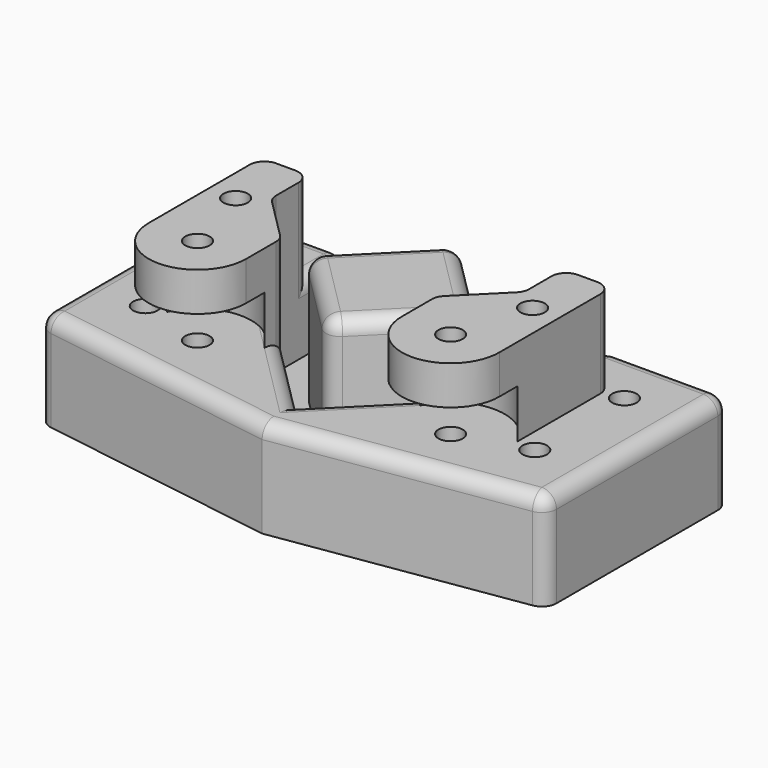
from build123d import *

# Parameters (mm, degrees)
F3_DEPTH      = 32
F0_R          = 2.5
F4_DEPTH      = 6
F5_DEPTH      = 20
F6_DEPTH      = 38
F2_R          = 11
F7_DEPTH      = 10
F8_T1_DEPTH   = 35.1066017178
F8_T3_DEPTH   = 18.6032957828
F8_T5_DEPTH   = 18.6032957828
F8_T7_DEPTH   = 18.6032957828
F8_T9_DEPTH   = 18.6032957828
F8_T11_DEPTH  = 23
F8_T13_DEPTH  = 21.1066017178
F8_T15_DEPTH  = 25.5
F8_T17_DEPTH  = 11
F8_T19_DEPTH  = 24.5
F8_T21_DEPTH  = 23.4343921757
F8_T23_DEPTH  = 7.1853823869
F8_T25_DEPTH  = 20
F8_T27_DEPTH  = 41.4262431297
F8_T29_DEPTH  = 62.7880288816
F8_T31_DEPTH  = 62.7880288816
F8_T33_DEPTH  = 20
F8_T35_DEPTH  = 52
F8_S39_W      = 3
F8_S39_H      = 3
F8_T40_DEPTH  = 3
F8_T46_DEPTH  = 3
F8_S51_W      = 3
F8_S51_H      = 3
F8_T52_DEPTH  = 3
F8_S57_W      = 3
F8_S57_H      = 3
F8_T58_DEPTH  = 3
F8_S63_W      = 3
F8_S63_H      = 3
F8_T64_DEPTH  = 3
F8_S69_W      = 3
F8_S69_H      = 3
F8_T70_DEPTH  = 3
F8_T76_DEPTH  = 3
F8_S81_W      = 3
F8_S81_H      = 3
F8_T82_DEPTH  = 3
F8_T88_DEPTH  = 3
F8_S93_W      = 3
F8_S93_H      = 3
F8_T94_DEPTH  = 3
F8_T100_DEPTH = 30.127416998
F8_S101_R     = 11
F8_T102_DEPTH = 18
F8_T107_DEPTH = 30.127416998
F8_T112_DEPTH = 30.127416998
F8_S113_R     = 11
F8_T114_DEPTH = 18
F8_T119_DEPTH = 30.127416998
F8_T124_DEPTH = 30.127416998
F8_S126_R     = 11
F8_T127_DEPTH = 18
F8_T131_DEPTH = 30.127416998
F8_S133_R     = 11
F8_T134_DEPTH = 18
F8_T139_DEPTH = 30.127416998
F8_S140_R     = 11
F8_T141_DEPTH = 18
F8_T145_DEPTH = 24.2132034356
F8_T152_DEPTH = 37.627416998
F8_T156_DEPTH = 37.627416998
F8_T163_DEPTH = 24.2132034356
F8_T167_DEPTH = 30.127416998
F8_S169_R     = 11
F8_T170_DEPTH = 18
F8_T176_DEPTH = 14.6853823869
F8_T180_DEPTH = 33
F8_T187_DEPTH = 33
F8_T191_DEPTH = 14.6853823869
F8_T198_DEPTH = 59.5
F8_T202_DEPTH = 18.5
F8_T209_DEPTH = 59.5
F8_T213_DEPTH = 18.5


# Not quite as in the source:
# - a fillet or chamfer that OpenCascade refuses, or shapes differently, is made with other operations: its cross-section is extruded or revolved along the edge and cut away or added


with BuildPart() as f3:
    # F0 (on Top) → F3 (new body)
    with BuildSketch(Plane.XY):
        Polygon((17.3971572875, -21.7171572875), (0, -4.32), (-17.3971572875, -21.7171572875), (0, -39.1143145751), align=None)
    extrude(amount=F3_DEPTH)

    # F0 (on Top) → F4 (join)
    with BuildSketch(Plane.XY):
        Polygon((26, 0), (0, 0), (-26, 0), (-26, -10.1853823869), (-26, -20.1853823869), (-16, -30.1853823869), (0, -46.1853823869), (16, -30.1853823869), (26, -20.1853823869), (26, -10.1853823869), align=None)
        with Locations((-21, -12)):
            Circle(F0_R, mode=Mode.SUBTRACT)
        Polygon((-17.3971572875, -21.7171572875), (0, -4.32), (17.3971572875, -21.7171572875), (0, -39.1143145751), align=None, mode=Mode.SUBTRACT)
        with Locations((21, -12)):
            Circle(F0_R, mode=Mode.SUBTRACT)
    extrude(amount=F4_DEPTH)

    # F0 (on Top) → F5 (join)
    with BuildSketch(Plane.XY):
        with BuildLine():
            Line((52, 0), (26, 0))
            Line((26, 0), (26, -10.1853823869))
            Line((26, -10.1853823869), (36, -10.1853823869))
            Line((36, -10.1853823869), (36, -39.1143145751))
            ThreePointArc((36, -39.1143145751), (26, -49.1143145751), (16, -39.1143145751))
            Line((16, -39.1143145751), (16, -30.1853823869))
            Line((16, -30.1853823869), (0, -46.1853823869))
            Line((0, -46.1853823869), (-16, -30.1853823869))
            Line((-16, -30.1853823869), (-16, -39.1143145751))
            ThreePointArc((-16, -39.1143145751), (-26, -49.1143145751), (-36, -39.1143145751))
            Line((-36, -39.1143145751), (-36, -10.1853823869))
            Line((-36, -10.1853823869), (-26, -10.1853823869))
            Line((-26, -10.1853823869), (-26, 0))
            Line((-26, 0), (-52, 0))
            Line((-52, 0), (-52, -47))
            Line((-52, -47), (0, -55))
            Line((0, -55), (52, -47))
            Line((52, -47), (52, 0))
        make_face()
        with Locations((-40, -35)):
            Circle(F0_R, mode=Mode.SUBTRACT)
        with Locations((40, -35)):
            Circle(F0_R, mode=Mode.SUBTRACT)
        with Locations((-40, -12)):
            Circle(F0_R, mode=Mode.SUBTRACT)
        with Locations((40, -12)):
            Circle(F0_R, mode=Mode.SUBTRACT)
    extrude(amount=F5_DEPTH)

    # F0 (on Top) → F6 (join)
    with BuildSketch(Plane.XY):
        with BuildLine():
            Line((-26, -20.1853823869), (-26, -10.1853823869))
            Line((-26, -10.1853823869), (-36, -10.1853823869))
            Line((-36, -10.1853823869), (-36, -39.1143145751))
            ThreePointArc((-36, -39.1143145751), (-26, -49.1143145751), (-16, -39.1143145751))
            Line((-16, -39.1143145751), (-16, -30.1853823869))
            Line((-16, -30.1853823869), (-26, -20.1853823869))
        make_face()
        with Locations((-26, -39.1143145751)):
            Circle(F0_R, mode=Mode.SUBTRACT)
        with Locations((-30.5, -23.6853823869)):
            Circle(F0_R, mode=Mode.SUBTRACT)
        with BuildLine():
            Line((36, -10.1853823869), (26, -10.1853823869))
            Line((26, -10.1853823869), (26, -20.1853823869))
            Line((26, -20.1853823869), (16, -30.1853823869))
            Line((16, -30.1853823869), (16, -39.1143145751))
            ThreePointArc((16, -39.1143145751), (26, -49.1143145751), (36, -39.1143145751))
            Line((36, -39.1143145751), (36, -10.1853823869))
        make_face()
        with Locations((26, -39.1143145751)):
            Circle(F0_R, mode=Mode.SUBTRACT)
        with Locations((30.5, -23.6853823869)):
            Circle(F0_R, mode=Mode.SUBTRACT)
    extrude(amount=F6_DEPTH)

    # F2 (on offset) → F7 (cut)
    with BuildSketch(Plane.XY.offset(20)):
        with Locations((-26, -39)):
            Circle(F2_R)
        with Locations((26, -39)):
            Circle(F2_R)
    extrude(amount=F7_DEPTH, mode=Mode.SUBTRACT)

    # F8: fillet of radius 3 on 33 edges, made by hand

    # F8_s2 → F8_t1 (join)
    with BuildSketch(Plane.XY.offset(2.8933982822)):
        with BuildLine():
            ThreePointArc((-26, -18.9427416998), (-25.7716385975, -20.0907919969), (-25.1213203436, -21.0640620434))
            Line((-25.1213203436, -21.0640620434), (-26, -20.1853823869))
            Line((-26, -20.1853823869), (-26, -18.9427416998))
        make_face()
        with BuildLine():
            ThreePointArc((25.1213203436, -21.0640620434), (25.7716385975, -20.0907919969), (26, -18.9427416998))
            Line((26, -18.9427416998), (26, -20.1853823869))
            Line((26, -20.1853823869), (25.1213203436, -21.0640620434))
        make_face()
    extrude(amount=F8_T1_DEPTH)

    # F8_s4 → F8_t3 (cut)
    with BuildSketch(Plane(origin=(4.2813203436, -4.2813203436, 0), x_dir=(0, 0, 1), z_dir=(0.7071067812, -0.7071067812, 0))):
        with BuildLine():
            ThreePointArc((32, 24.6579970775), (31.1213203436, 26.779317421), (29, 27.6579970775))
            Line((29, 27.6579970775), (32, 27.6579970775))
            Line((32, 27.6579970775), (32, 24.6579970775))
        make_face()
    extrude(amount=F8_T3_DEPTH, mode=Mode.SUBTRACT)

    # F8_s6 → F8_t5 (cut)
    with BuildSketch(Plane(origin=(17.435836944, -17.435836944, 0), x_dir=(0, 0, 1), z_dir=(-0.7071067812, 0.7071067812, 0))):
        with BuildLine():
            ThreePointArc((29, -3.0547012947), (31.1213203436, -3.9333809512), (32, -6.0547012947))
            Line((32, -6.0547012947), (32, -3.0547012947))
            Line((32, -3.0547012947), (29, -3.0547012947))
        make_face()
    extrude(amount=F8_T5_DEPTH, mode=Mode.SUBTRACT)

    # F8_s8 → F8_t7 (cut)
    with BuildSketch(Plane(origin=(-4.2813203436, -4.2813203436, 0), x_dir=(0, 0, 1), z_dir=(-0.7071067812, -0.7071067812, 0))):
        with BuildLine():
            ThreePointArc((29, -3.0547012947), (31.1213203436, -3.9333809512), (32, -6.0547012947))
            Line((32, -6.0547012947), (32, -3.0547012947))
            Line((32, -3.0547012947), (29, -3.0547012947))
        make_face()
    extrude(amount=F8_T7_DEPTH, mode=Mode.SUBTRACT)

    # F8_s10 → F8_t9 (cut)
    with BuildSketch(Plane(origin=(-17.435836944, -17.435836944, 0), x_dir=(0, 0, 1), z_dir=(0.7071067812, 0.7071067812, 0))):
        with BuildLine():
            ThreePointArc((32, 24.6579970775), (31.1213203436, 26.779317421), (29, 27.6579970775))
            Line((29, 27.6579970775), (32, 27.6579970775))
            Line((32, 27.6579970775), (32, 24.6579970775))
        make_face()
    extrude(amount=F8_T9_DEPTH, mode=Mode.SUBTRACT)

    # F8_s12 → F8_t11 (cut)
    with BuildSketch(Plane.XY.offset(6)):
        with BuildLine():
            ThreePointArc((2.1213203436, -36.9929942315), (0, -37.8716738879), (-2.1213203436, -36.9929942315))
            Line((-2.1213203436, -36.9929942315), (0, -39.1143145751))
            Line((0, -39.1143145751), (2.1213203436, -36.9929942315))
        make_face()
        with BuildLine():
            ThreePointArc((15.275836944, -19.595836944), (16.1545166004, -21.7171572875), (15.275836944, -23.8384776311))
            Line((15.275836944, -23.8384776311), (17.3971572875, -21.7171572875))
            Line((17.3971572875, -21.7171572875), (15.275836944, -19.595836944))
        make_face()
        with BuildLine():
            ThreePointArc((2.1213203436, -6.4413203436), (0, -5.5626406871), (-2.1213203436, -6.4413203436))
            Line((-2.1213203436, -6.4413203436), (0, -4.32))
            Line((0, -4.32), (2.1213203436, -6.4413203436))
        make_face()
        with BuildLine():
            ThreePointArc((-15.275836944, -19.595836944), (-16.1545166004, -21.7171572875), (-15.275836944, -23.8384776311))
            Line((-15.275836944, -23.8384776311), (-17.3971572875, -21.7171572875))
            Line((-17.3971572875, -21.7171572875), (-15.275836944, -19.595836944))
        make_face()
    extrude(amount=F8_T11_DEPTH, mode=Mode.SUBTRACT)

    # F8_s14 → F8_t13 (cut)
    with BuildSketch(Plane.XY.offset(20)):
        with BuildLine():
            ThreePointArc((16.8786796564, -29.3067027305), (16.2283614025, -30.2799727769), (16, -31.428023074))
            Line((16, -31.428023074), (16, -30.1853823869))
            Line((16, -30.1853823869), (16.8786796564, -29.3067027305))
        make_face()
        with BuildLine():
            ThreePointArc((-16.8786796564, -29.3067027305), (-16.2283614025, -30.2799727769), (-16, -31.428023074))
            Line((-16, -31.428023074), (-16, -30.1853823869))
            Line((-16, -30.1853823869), (-16.8786796564, -29.3067027305))
        make_face()
    extrude(amount=F8_T13_DEPTH, mode=Mode.SUBTRACT)

    # F8_s16 → F8_t15 (cut)
    with BuildSketch(Plane.XY.offset(20)):
        with BuildLine():
            ThreePointArc((-26, -13.1853823869), (-26.8786796564, -11.0640620434), (-29, -10.1853823869))
            Line((-29, -10.1853823869), (-26, -10.1853823869))
            Line((-26, -10.1853823869), (-26, -13.1853823869))
        make_face()
        with BuildLine():
            ThreePointArc((26, -13.1853823869), (26.8786796564, -11.0640620434), (29, -10.1853823869))
            Line((29, -10.1853823869), (26, -10.1853823869))
            Line((26, -10.1853823869), (26, -13.1853823869))
        make_face()
        with BuildLine():
            ThreePointArc((-33, -10.1853823869), (-35.1213203436, -11.0640620434), (-36, -13.1853823869))
            Line((-36, -13.1853823869), (-36, -10.1853823869))
            Line((-36, -10.1853823869), (-33, -10.1853823869))
        make_face()
        with BuildLine():
            ThreePointArc((33, -10.1853823869), (35.1213203436, -11.0640620434), (36, -13.1853823869))
            Line((36, -13.1853823869), (36, -10.1853823869))
            Line((36, -10.1853823869), (33, -10.1853823869))
        make_face()
    extrude(amount=F8_T15_DEPTH, mode=Mode.SUBTRACT)

    # F8_s18 → F8_t17 (cut)
    with BuildSketch(Plane.XY.offset(6)):
        with BuildLine():
            ThreePointArc((29, 0), (26.8786796564, -0.8786796564), (26, -3))
            Line((26, -3), (26, 0))
            Line((26, 0), (29, 0))
        make_face()
        with BuildLine():
            ThreePointArc((-29, 0), (-26.8786796564, -0.8786796564), (-26, -3))
            Line((-26, -3), (-26, 0))
            Line((-26, 0), (-29, 0))
        make_face()
    extrude(amount=F8_T17_DEPTH, mode=Mode.SUBTRACT)

    # F8_s20 → F8_t19 (cut)
    with BuildSketch(Plane.XY.offset(-7.5)):
        with BuildLine():
            ThreePointArc((-49, 0), (-51.1213203436, -0.8786796564), (-52, -3))
            Line((-52, -3), (-52, 0))
            Line((-52, 0), (-49, 0))
        make_face()
        with BuildLine():
            ThreePointArc((49, 0), (51.1213203436, -0.8786796564), (52, -3))
            Line((52, -3), (52, 0))
            Line((52, 0), (49, 0))
        make_face()
    extrude(amount=F8_T19_DEPTH, mode=Mode.SUBTRACT)

    # F8_s22 → F8_t21 (cut)
    with BuildSketch(Plane.XY.offset(-6.4343921757)):
        with BuildLine():
            ThreePointArc((-52, -44.4262431297), (-51.2768964248, -46.3796357351), (-49.4561715528, -47.3913582227))
            Line((-49.4561715528, -47.3913582227), (-52, -47))
            Line((-52, -47), (-52, -44.4262431297))
        make_face()
        with BuildLine():
            ThreePointArc((52, -44.4262431297), (51.2768964248, -46.3796357351), (49.4561715528, -47.3913582227))
            Line((49.4561715528, -47.3913582227), (52, -47))
            Line((52, -47), (52, -44.4262431297))
        make_face()
    extrude(amount=F8_T21_DEPTH, mode=Mode.SUBTRACT)

    # F8_s24 → F8_t23 (cut)
    with BuildSketch(Plane.XZ.offset(3)):
        with BuildLine():
            ThreePointArc((26, 17), (26.8786796564, 19.1213203436), (29, 20))
            Line((29, 20), (26, 20))
            Line((26, 20), (26, 17))
        make_face()
        with BuildLine():
            ThreePointArc((-26, 17), (-26.8786796564, 19.1213203436), (-29, 20))
            Line((-29, 20), (-26, 20))
            Line((-26, 20), (-26, 17))
        make_face()
    extrude(amount=F8_T23_DEPTH, mode=Mode.SUBTRACT)

    # F8_s26 → F8_t25 (cut)
    with BuildSketch(Plane.YZ.offset(29)):
        with BuildLine():
            ThreePointArc((0, 17), (-0.8786796564, 19.1213203436), (-3, 20))
            Line((-3, 20), (0, 20))
            Line((0, 20), (0, 17))
        make_face()
    extrude(amount=F8_T25_DEPTH, mode=Mode.SUBTRACT)

    # F8_s28 → F8_t27 (cut)
    with BuildSketch(Plane.XZ.offset(3)):
        with BuildLine():
            ThreePointArc((49, 20), (51.1213203436, 19.1213203436), (52, 17))
            Line((52, 17), (52, 20))
            Line((52, 20), (49, 20))
        make_face()
        with BuildLine():
            ThreePointArc((-49, 20), (-51.1213203436, 19.1213203436), (-52, 17))
            Line((-52, 17), (-52, 20))
            Line((-52, 20), (-49, 20))
        make_face()
    extrude(amount=F8_T27_DEPTH, mode=Mode.SUBTRACT)

    # F8_s30 → F8_t29 (cut)
    with BuildSketch(Plane(origin=(-20.8676350988, -3.2104053998, 0), x_dir=(0, 0, 1), z_dir=(0.9883716977, 0.1520571843, 0))):
        with BuildLine():
            ThreePointArc((20, 51.3604433708), (19.1213203436, 53.4817637143), (17, 54.3604433708))
            Line((17, 54.3604433708), (20, 54.3604433708))
            Line((20, 54.3604433708), (20, 51.3604433708))
        make_face()
    extrude(amount=F8_T29_DEPTH, mode=Mode.SUBTRACT)

    # F8_s32 → F8_t31 (cut)
    with BuildSketch(Plane(origin=(-41.190275599, 6.3369654768, 0), x_dir=(0, 0, 1), z_dir=(0.9883716977, -0.1520571843, 0))):
        with BuildLine():
            ThreePointArc((20, 51.3604433708), (19.1213203436, 53.4817637143), (17, 54.3604433708))
            Line((17, 54.3604433708), (20, 54.3604433708))
            Line((20, 54.3604433708), (20, 51.3604433708))
        make_face()
    extrude(amount=F8_T31_DEPTH, mode=Mode.SUBTRACT)

    # F8_s34 → F8_t33 (cut)
    with BuildSketch(Plane.YZ.offset(-49)):
        with BuildLine():
            ThreePointArc((0, 17), (-0.8786796564, 19.1213203436), (-3, 20))
            Line((-3, 20), (0, 20))
            Line((0, 20), (0, 17))
        make_face()
    extrude(amount=F8_T33_DEPTH, mode=Mode.SUBTRACT)

    # F8_s36 → F8_t35 (cut)
    with BuildSketch(Plane.YZ.offset(-26)):
        with BuildLine():
            ThreePointArc((-3, 6), (-0.8786796564, 5.1213203436), (0, 3))
            Line((0, 3), (0, 6))
            Line((0, 6), (-3, 6))
        make_face()
    extrude(amount=F8_T35_DEPTH, mode=Mode.SUBTRACT)


with BuildPart() as f8_tool38:
    # F8_s39 → F8_t40 (new body)
    with BuildSketch(Plane(origin=(4.2813203436, -4.2813203436, 0), x_dir=(0, 0, 1), z_dir=(-0.7071067812, 0.7071067812, 0))):
        with Locations((30.5, -26.1579970775)):
            Rectangle(F8_S39_W, F8_S39_H)
    extrude(amount=F8_T40_DEPTH)

    # F8_s41 → F8_t42 (revolve, cut)
    with BuildSketch(Plane(origin=(-13.1545166004, -21.7171572875, 29), x_dir=(0.5, 0.5, -0.7071067812), z_dir=(0.5, 0.5, 0.7071067812))):
        with BuildLine():
            ThreePointArc((0, -3), (3, 0), (0, 3))
            Line((0, 3), (0, -3))
        make_face()
    revolve(axis=Axis((-13.1545166004, -21.7171572875, 29), (-0.7071067812, 0.7071067812, 0)), mode=Mode.SUBTRACT)


with BuildPart() as f3_1:
    add(f3.part)

    # F8_t37: cut F8_tool38
    add(f8_tool38.part, mode=Mode.SUBTRACT)


with BuildPart() as f8_tool44:
    # F8_s45 → F8_t46 (new body)
    with BuildSketch(Plane.XY.offset(29)):
        Polygon((0, -34.8716738879), (2.1213203436, -36.9929942315), (0, -39.1143145751), (-2.1213203436, -36.9929942315), align=None)
    extrude(amount=F8_T46_DEPTH)

    # F8_s47 → F8_t48 (revolve, cut)
    with BuildSketch(Plane(origin=(0, -34.8716738879, 29), x_dir=(0, 1, 0), z_dir=(1, 0, 0))):
        with BuildLine():
            ThreePointArc((0, -3), (3, 0), (0, 3))
            Line((0, 3), (0, -3))
        make_face()
    revolve(axis=Axis((0, -34.8716738879, 29), (0, 0, 1)), mode=Mode.SUBTRACT)


with BuildPart() as f3_2:
    add(f3_1.part)

    # F8_t43: cut F8_tool44
    add(f8_tool44.part, mode=Mode.SUBTRACT)


with BuildPart() as f8_tool50:
    # F8_s51 → F8_t52 (new body)
    with BuildSketch(Plane(origin=(-4.2813203436, -4.2813203436, 0), x_dir=(0, 0, 1), z_dir=(0.7071067812, 0.7071067812, 0))):
        with Locations((30.5, 26.1579970775)):
            Rectangle(F8_S51_W, F8_S51_H)
    extrude(amount=F8_T52_DEPTH)

    # F8_s53 → F8_t54 (revolve, cut)
    with BuildSketch(Plane(origin=(13.1545166004, -21.7171572875, 29), x_dir=(-0.5, 0.5, -0.7071067812), z_dir=(0.5, -0.5, -0.7071067812))):
        with BuildLine():
            ThreePointArc((0, -3), (3, 0), (0, 3))
            Line((0, 3), (0, -3))
        make_face()
    revolve(axis=Axis((13.1545166004, -21.7171572875, 29), (0.7071067812, 0.7071067812, 0)), mode=Mode.SUBTRACT)


with BuildPart() as f3_3:
    add(f3_2.part)

    # F8_t49: cut F8_tool50
    add(f8_tool50.part, mode=Mode.SUBTRACT)


with BuildPart() as f8_tool56:
    # F8_s57 → F8_t58 (new body)
    with BuildSketch(Plane(origin=(-4.2813203436, -4.2813203436, 0), x_dir=(0, 0, 1), z_dir=(0.7071067812, 0.7071067812, 0))):
        with Locations((30.5, 4.5547012947)):
            Rectangle(F8_S57_W, F8_S57_H)
    extrude(amount=F8_T58_DEPTH)

    # F8_s59 → F8_t60 (revolve, cut)
    with BuildSketch(Plane(origin=(0, -8.5626406871, 29), x_dir=(0.5, -0.5, -0.7071067812), z_dir=(0.5, -0.5, 0.7071067812))):
        with BuildLine():
            ThreePointArc((0, -3), (3, 0), (0, 3))
            Line((0, 3), (0, -3))
        make_face()
    revolve(axis=Axis((0, -8.5626406871, 29), (0.7071067812, 0.7071067812, 0)), mode=Mode.SUBTRACT)


with BuildPart() as f3_4:
    add(f3_3.part)

    # F8_t55: cut F8_tool56
    add(f8_tool56.part, mode=Mode.SUBTRACT)


with BuildPart() as f8_tool62:
    # F8_s63 → F8_t64 (new body)
    with BuildSketch(Plane.XZ.offset(3)):
        with Locations((27.5, 18.5)):
            Rectangle(F8_S63_W, F8_S63_H)
    extrude(amount=-F8_T64_DEPTH)

    # F8_s65 → F8_t66 (revolve, cut)
    with BuildSketch(Plane(origin=(29, -3, 17), x_dir=(0.7071067812, 0, -0.7071067812), z_dir=(0.7071067812, 0, 0.7071067812))):
        with BuildLine():
            ThreePointArc((0, -3), (3, 0), (0, 3))
            Line((0, 3), (0, -3))
        make_face()
    revolve(axis=Axis((29, -3, 17), (0, 1, 0)), mode=Mode.SUBTRACT)


with BuildPart() as f3_5:
    add(f3_4.part)

    # F8_t61: cut F8_tool62
    add(f8_tool62.part, mode=Mode.SUBTRACT)


with BuildPart() as f8_tool68:
    # F8_s69 → F8_t70 (new body)
    with BuildSketch(Plane.YZ.offset(-49)):
        with Locations((-1.5, 18.5)):
            Rectangle(F8_S69_W, F8_S69_H)
    extrude(amount=-F8_T70_DEPTH)

    # F8_s71 → F8_t72 (revolve, cut)
    with BuildSketch(Plane(origin=(-49, -3, 17), x_dir=(0, -0.7071067812, -0.7071067812), z_dir=(0, 0.7071067812, -0.7071067812))):
        with BuildLine():
            ThreePointArc((0, -3), (3, 0), (0, 3))
            Line((0, 3), (0, -3))
        make_face()
    revolve(axis=Axis((-49, -3, 17), (-1, 0, 0)), mode=Mode.SUBTRACT)


with BuildPart() as f3_6:
    add(f3_5.part)

    # F8_t67: cut F8_tool68
    add(f8_tool68.part, mode=Mode.SUBTRACT)


with BuildPart() as f8_tool74:
    # F8_s75 → F8_t76 (new body)
    with BuildSketch(Plane.XY.offset(17)):
        Polygon((-49, -44.4262431297), (-52, -44.4262431297), (-52, -47), (-49.4561715528, -47.3913582227), align=None)
    extrude(amount=F8_T76_DEPTH)

    # F8_s77 → F8_t78 (revolve, cut)
    with BuildSketch(Plane(origin=(-49, -44.4262431297, 17), x_dir=(0.7589654749, 0.6511308685, 0), z_dir=(0.6511308685, -0.7589654749, 0))):
        with BuildLine():
            ThreePointArc((0, -3), (3, 0), (0, 3))
            Line((0, 3), (0, -3))
        make_face()
    revolve(axis=Axis((-49, -44.4262431297, 17), (0, 0, 1)), mode=Mode.SUBTRACT)


with BuildPart() as f3_7:
    add(f3_6.part)

    # F8_t73: cut F8_tool74
    add(f8_tool74.part, mode=Mode.SUBTRACT)


with BuildPart() as f8_tool80:
    # F8_s81 → F8_t82 (new body)
    with BuildSketch(Plane.YZ.offset(49)):
        with Locations((-1.5, 18.5)):
            Rectangle(F8_S81_W, F8_S81_H)
    extrude(amount=F8_T82_DEPTH)

    # F8_s83 → F8_t84 (revolve, cut)
    with BuildSketch(Plane(origin=(49, -3, 17), x_dir=(0, -0.7071067812, -0.7071067812), z_dir=(0, -0.7071067812, 0.7071067812))):
        with BuildLine():
            ThreePointArc((0, -3), (3, 0), (0, 3))
            Line((0, 3), (0, -3))
        make_face()
    revolve(axis=Axis((49, -3, 17), (1, 0, 0)), mode=Mode.SUBTRACT)


with BuildPart() as f3_8:
    add(f3_7.part)

    # F8_t79: cut F8_tool80
    add(f8_tool80.part, mode=Mode.SUBTRACT)


with BuildPart() as f8_tool86:
    # F8_s87 → F8_t88 (new body)
    with BuildSketch(Plane.XY.offset(17)):
        Polygon((49, -44.4262431297), (52, -44.4262431297), (52, -47), (49.4561715528, -47.3913582227), align=None)
    extrude(amount=F8_T88_DEPTH)

    # F8_s89 → F8_t90 (revolve, cut)
    with BuildSketch(Plane(origin=(49, -44.4262431297, 17), x_dir=(-0.7589654749, 0.6511308685, 0), z_dir=(0.6511308685, 0.7589654749, 0))):
        with BuildLine():
            ThreePointArc((0, -3), (3, 0), (0, 3))
            Line((0, 3), (0, -3))
        make_face()
    revolve(axis=Axis((49, -44.4262431297, 17), (0, 0, 1)), mode=Mode.SUBTRACT)


with BuildPart() as f3_9:
    add(f3_8.part)

    # F8_t85: cut F8_tool86
    add(f8_tool86.part, mode=Mode.SUBTRACT)


with BuildPart() as f8_tool92:
    # F8_s93 → F8_t94 (new body)
    with BuildSketch(Plane.YZ.offset(-29)):
        with Locations((-1.5, 18.5)):
            Rectangle(F8_S93_W, F8_S93_H)
    extrude(amount=F8_T94_DEPTH)

    # F8_s95 → F8_t96 (revolve, cut)
    with BuildSketch(Plane(origin=(-29, -3, 17), x_dir=(0, -0.7071067812, -0.7071067812), z_dir=(0, -0.7071067812, 0.7071067812))):
        with BuildLine():
            ThreePointArc((0, -3), (3, 0), (0, 3))
            Line((0, 3), (0, -3))
        make_face()
    revolve(axis=Axis((-29, -3, 17), (1, 0, 0)), mode=Mode.SUBTRACT)


with BuildPart() as f3_10:
    add(f3_9.part)

    # F8_t91: cut F8_tool92
    add(f8_tool92.part, mode=Mode.SUBTRACT)


with BuildPart() as f8_tool98:
    # F8_s99 → F8_t100 (new body)
    with BuildSketch(Plane(origin=(-1.7893903346, -1.7893903346, 0), x_dir=(0, 0, 1), z_dir=(-0.7071067812, -0.7071067812, 0))):
        with BuildLine():
            ThreePointArc((17, -32.6579970775), (19.1213203436, -33.5366767339), (20, -35.6579970775))
            Line((20, -35.6579970775), (20, -32.6579970775))
            Line((20, -32.6579970775), (17, -32.6579970775))
        make_face()
    extrude(amount=F8_T100_DEPTH)

    # F8_s101 → F8_t102 (intersect, symmetric)
    with BuildSketch(Plane.XY.offset(18.5)):
        with Locations((26, -39)):
            Circle(F8_S101_R)
    extrude(amount=F8_T102_DEPTH, both=True, mode=Mode.INTERSECT)

    split(bisect_by=Plane.YZ.offset(16), keep=Keep.TOP)


with BuildPart() as f3_11:
    add(f3_10.part)

    # F8_t97: cut F8_tool98
    add(f8_tool98.part, mode=Mode.SUBTRACT)


with BuildPart() as f8_tool105:
    # F8_s106 → F8_t107 (new body)
    with BuildSketch(Plane(origin=(-1.7893903346, -1.7893903346, 0), x_dir=(0, 0, 1), z_dir=(-0.7071067812, -0.7071067812, 0))):
        with BuildLine():
            ThreePointArc((17, -32.6579970775), (19.1213203436, -33.5366767339), (20, -35.6579970775))
            Line((20, -35.6579970775), (20, -32.6579970775))
            Line((20, -32.6579970775), (17, -32.6579970775))
        make_face()
    extrude(amount=F8_T107_DEPTH)

    split(bisect_by=Plane.YZ.offset(16), keep=Keep.BOTTOM)


with BuildPart() as f3_12:
    add(f3_11.part)

    # F8_t104: cut F8_tool105
    add(f8_tool105.part, mode=Mode.SUBTRACT)


with BuildPart() as f8_tool110:
    # F8_s111 → F8_t112 (new body)
    with BuildSketch(Plane(origin=(-1.7893903346, -1.7893903346, 0), x_dir=(0, 0, 1), z_dir=(-0.7071067812, -0.7071067812, 0))):
        with BuildLine():
            ThreePointArc((17, -32.6579970775), (19.1213203436, -33.5366767339), (20, -35.6579970775))
            Line((20, -35.6579970775), (20, -32.6579970775))
            Line((20, -32.6579970775), (17, -32.6579970775))
        make_face()
    extrude(amount=F8_T112_DEPTH)

    # F8_s113 → F8_t114 (intersect, symmetric)
    with BuildSketch(Plane.XY.offset(18.5)):
        with Locations((26, -39)):
            Circle(F8_S113_R)
    extrude(amount=F8_T114_DEPTH, both=True, mode=Mode.INTERSECT)

    split(bisect_by=Plane.YZ.offset(16), keep=Keep.BOTTOM)


with BuildPart() as f3_13:
    add(f3_12.part)

    # F8_t109: cut F8_tool110
    add(f8_tool110.part, mode=Mode.SUBTRACT)


with BuildPart() as f8_tool117:
    # F8_s118 → F8_t119 (new body)
    with BuildSketch(Plane(origin=(23.0926911935, -23.0926911935, 0), x_dir=(0, 0, 1), z_dir=(-0.7071067812, 0.7071067812, 0))):
        with BuildLine():
            ThreePointArc((17, -32.6579970775), (19.1213203436, -33.5366767339), (20, -35.6579970775))
            Line((20, -35.6579970775), (20, -32.6579970775))
            Line((20, -32.6579970775), (17, -32.6579970775))
        make_face()
    extrude(amount=F8_T119_DEPTH)

    split(bisect_by=Plane.YZ.offset(-16), keep=Keep.TOP)


with BuildPart() as f3_14:
    add(f3_13.part)

    # F8_t116: cut F8_tool117
    add(f8_tool117.part, mode=Mode.SUBTRACT)


with BuildPart() as f8_tool122:
    # F8_s123 → F8_t124 (new body)
    with BuildSketch(Plane(origin=(23.0926911935, -23.0926911935, 0), x_dir=(0, 0, 1), z_dir=(-0.7071067812, 0.7071067812, 0))):
        with BuildLine():
            ThreePointArc((17, -32.6579970775), (19.1213203436, -33.5366767339), (20, -35.6579970775))
            Line((20, -35.6579970775), (20, -32.6579970775))
            Line((20, -32.6579970775), (17, -32.6579970775))
        make_face()
    extrude(amount=F8_T124_DEPTH)

    split(bisect_by=Plane.YZ.offset(-16), keep=Keep.TOP)

    # F8_s126 → F8_t127 (intersect, symmetric)
    with BuildSketch(Plane.XY.offset(18.5)):
        with Locations((-26, -39)):
            Circle(F8_S126_R)
    extrude(amount=F8_T127_DEPTH, both=True, mode=Mode.INTERSECT)


with BuildPart() as f3_15:
    add(f3_14.part)

    # F8_t121: cut F8_tool122
    add(f8_tool122.part, mode=Mode.SUBTRACT)


with BuildPart() as f8_tool129:
    # F8_s130 → F8_t131 (new body)
    with BuildSketch(Plane(origin=(23.0926911935, -23.0926911935, 0), x_dir=(0, 0, 1), z_dir=(-0.7071067812, 0.7071067812, 0))):
        with BuildLine():
            ThreePointArc((17, -32.6579970775), (19.1213203436, -33.5366767339), (20, -35.6579970775))
            Line((20, -35.6579970775), (20, -32.6579970775))
            Line((20, -32.6579970775), (17, -32.6579970775))
        make_face()
    extrude(amount=F8_T131_DEPTH)

    split(bisect_by=Plane.YZ.offset(-16), keep=Keep.BOTTOM)

    # F8_s133 → F8_t134 (intersect, symmetric)
    with BuildSketch(Plane.XY.offset(18.5)):
        with Locations((-26, -39)):
            Circle(F8_S133_R)
    extrude(amount=F8_T134_DEPTH, both=True, mode=Mode.INTERSECT)


with BuildPart() as f3_16:
    add(f3_15.part)

    # F8_t128: cut F8_tool129
    add(f8_tool129.part, mode=Mode.SUBTRACT)


with BuildPart() as f8_tool137:
    # F8_s138 → F8_t139 (new body)
    with BuildSketch(Plane(origin=(-1.7893903346, -1.7893903346, 0), x_dir=(0, 0, 1), z_dir=(-0.7071067812, -0.7071067812, 0))):
        with BuildLine():
            ThreePointArc((17, -32.6579970775), (19.1213203436, -33.5366767339), (20, -35.6579970775))
            Line((20, -35.6579970775), (20, -32.6579970775))
            Line((20, -32.6579970775), (17, -32.6579970775))
        make_face()
    extrude(amount=F8_T139_DEPTH)

    # F8_s140 → F8_t141 (cut, symmetric)
    with BuildSketch(Plane.XY.offset(18.5)):
        with Locations((26, -39)):
            Circle(F8_S140_R)
    extrude(amount=F8_T141_DEPTH, both=True, mode=Mode.SUBTRACT)

    split(bisect_by=Plane.YZ.offset(16), keep=Keep.TOP)


with BuildPart() as f8_tool143:
    # F8_s144 → F8_t145 (new body)
    with BuildSketch(Plane.XY.offset(16.8933982822)):
        with BuildLine():
            ThreePointArc((16.8786796564, -29.3067027305), (16.2283614025, -30.2799727769), (16, -31.428023074))
            Line((16, -31.428023074), (16, -30.1853823869))
            Line((16, -30.1853823869), (16.8786796564, -29.3067027305))
        make_face()
    extrude(amount=F8_T145_DEPTH)

    split(bisect_by=Plane.XY.offset(20), keep=Keep.BOTTOM)


with BuildPart() as f8_tool137_1:
    add(f8_tool137.part)

    # F8_t147: intersect F8_tool143
    add(f8_tool143.part, mode=Mode.INTERSECT)


with BuildPart() as f3_17:
    add(f3_16.part)

    # F8_t135: cut F8_tool137
    add(f8_tool137_1.part, mode=Mode.SUBTRACT)


with BuildPart() as f8_tool150:
    # F8_s151 → F8_t152 (new body)
    with BuildSketch(Plane(origin=(-1.7893903346, -1.7893903346, 0), x_dir=(0, 0, 1), z_dir=(-0.7071067812, -0.7071067812, 0))):
        with BuildLine():
            ThreePointArc((17, -32.6579970775), (19.1213203436, -33.5366767339), (20, -35.6579970775))
            Line((20, -35.6579970775), (20, -32.6579970775))
            Line((20, -32.6579970775), (17, -32.6579970775))
        make_face()
    extrude(amount=F8_T152_DEPTH)

    split(bisect_by=Plane(origin=(-23.0926911935, -23.0926911935, 0), x_dir=(0, 0, 1), z_dir=(-0.7071067812, -0.7071067812, 0)), keep=Keep.TOP)


with BuildPart() as f8_tool154:
    # F8_s155 → F8_t156 (new body)
    with BuildSketch(Plane(origin=(28.3959920524, -28.3959920524, 0), x_dir=(0, 0, 1), z_dir=(-0.7071067812, 0.7071067812, 0))):
        with BuildLine():
            ThreePointArc((17, -32.6579970775), (19.1213203436, -33.5366767339), (20, -35.6579970775))
            Line((20, -35.6579970775), (20, -32.6579970775))
            Line((20, -32.6579970775), (17, -32.6579970775))
        make_face()
    extrude(amount=F8_T156_DEPTH)

    split(bisect_by=Plane(origin=(23.0926911935, -23.0926911935, 0), x_dir=(0, 0, 1), z_dir=(0.7071067812, -0.7071067812, 0)), keep=Keep.TOP)


with BuildPart() as f8_tool150_1:
    add(f8_tool150.part)

    # F8_t158: intersect F8_tool154
    add(f8_tool154.part, mode=Mode.INTERSECT)


with BuildPart() as f3_18:
    add(f3_17.part)

    # F8_t148: cut F8_tool150
    add(f8_tool150_1.part, mode=Mode.SUBTRACT)


with BuildPart() as f8_tool161:
    # F8_s162 → F8_t163 (new body)
    with BuildSketch(Plane.XY.offset(16.8933982822)):
        with BuildLine():
            ThreePointArc((-16.8786796564, -29.3067027305), (-16.2283614025, -30.2799727769), (-16, -31.428023074))
            Line((-16, -31.428023074), (-16, -30.1853823869))
            Line((-16, -30.1853823869), (-16.8786796564, -29.3067027305))
        make_face()
    extrude(amount=F8_T163_DEPTH)

    split(bisect_by=Plane.XY.offset(20), keep=Keep.BOTTOM)


with BuildPart() as f8_tool165:
    # F8_s166 → F8_t167 (new body)
    with BuildSketch(Plane(origin=(23.0926911935, -23.0926911935, 0), x_dir=(0, 0, 1), z_dir=(-0.7071067812, 0.7071067812, 0))):
        with BuildLine():
            ThreePointArc((17, -32.6579970775), (19.1213203436, -33.5366767339), (20, -35.6579970775))
            Line((20, -35.6579970775), (20, -32.6579970775))
            Line((20, -32.6579970775), (17, -32.6579970775))
        make_face()
    extrude(amount=F8_T167_DEPTH)

    split(bisect_by=Plane.YZ.offset(-16), keep=Keep.BOTTOM)

    # F8_s169 → F8_t170 (cut, symmetric)
    with BuildSketch(Plane.XY.offset(18.5)):
        with Locations((-26, -39)):
            Circle(F8_S169_R)
    extrude(amount=F8_T170_DEPTH, both=True, mode=Mode.SUBTRACT)


with BuildPart() as f8_tool161_1:
    add(f8_tool161.part)

    # F8_t171: intersect F8_tool165
    add(f8_tool165.part, mode=Mode.INTERSECT)


with BuildPart() as f3_19:
    add(f3_18.part)

    # F8_t159: cut F8_tool161
    add(f8_tool161_1.part, mode=Mode.SUBTRACT)


with BuildPart() as f8_tool174:
    # F8_s175 → F8_t176 (new body)
    with BuildSketch(Plane.XZ.offset(17.6853823869)):
        with BuildLine():
            ThreePointArc((-26, 17), (-26.8786796564, 19.1213203436), (-29, 20))
            Line((-29, 20), (-26, 20))
            Line((-26, 20), (-26, 17))
        make_face()
    extrude(amount=-F8_T176_DEPTH)

    split(bisect_by=Plane.XZ.offset(10.1853823869), keep=Keep.TOP)


with BuildPart() as f8_tool178:
    # F8_s179 → F8_t180 (new body)
    with BuildSketch(Plane.XY.offset(12.5)):
        with BuildLine():
            ThreePointArc((-26, -13.1853823869), (-26.8786796564, -11.0640620434), (-29, -10.1853823869))
            Line((-29, -10.1853823869), (-26, -10.1853823869))
            Line((-26, -10.1853823869), (-26, -13.1853823869))
        make_face()
    extrude(amount=F8_T180_DEPTH)

    split(bisect_by=Plane.XY.offset(20), keep=Keep.BOTTOM)


with BuildPart() as f8_tool174_1:
    add(f8_tool174.part)

    # F8_t182: intersect F8_tool178
    add(f8_tool178.part, mode=Mode.INTERSECT)


with BuildPart() as f3_20:
    add(f3_19.part)

    # F8_t172: cut F8_tool174
    add(f8_tool174_1.part, mode=Mode.SUBTRACT)


with BuildPart() as f8_tool185:
    # F8_s186 → F8_t187 (new body)
    with BuildSketch(Plane.XY.offset(12.5)):
        with BuildLine():
            ThreePointArc((26, -13.1853823869), (26.8786796564, -11.0640620434), (29, -10.1853823869))
            Line((29, -10.1853823869), (26, -10.1853823869))
            Line((26, -10.1853823869), (26, -13.1853823869))
        make_face()
    extrude(amount=F8_T187_DEPTH)

    split(bisect_by=Plane.XY.offset(20), keep=Keep.BOTTOM)


with BuildPart() as f8_tool189:
    # F8_s190 → F8_t191 (new body)
    with BuildSketch(Plane.XZ.offset(3)):
        with BuildLine():
            ThreePointArc((26, 17), (26.8786796564, 19.1213203436), (29, 20))
            Line((29, 20), (26, 20))
            Line((26, 20), (26, 17))
        make_face()
    extrude(amount=F8_T191_DEPTH)

    split(bisect_by=Plane.XZ.offset(10.1853823869), keep=Keep.TOP)


with BuildPart() as f8_tool185_1:
    add(f8_tool185.part)

    # F8_t193: intersect F8_tool189
    add(f8_tool189.part, mode=Mode.INTERSECT)


with BuildPart() as f3_21:
    add(f3_20.part)

    # F8_t183: cut F8_tool185
    add(f8_tool185_1.part, mode=Mode.SUBTRACT)


with BuildPart() as f8_tool196:
    # F8_s197 → F8_t198 (new body)
    with BuildSketch(Plane.YZ.offset(-26)):
        with BuildLine():
            ThreePointArc((-3, 6), (-0.8786796564, 5.1213203436), (0, 3))
            Line((0, 3), (0, 6))
            Line((0, 6), (-3, 6))
        make_face()
    extrude(amount=F8_T198_DEPTH)

    split(bisect_by=Plane.YZ.offset(26), keep=Keep.TOP)


with BuildPart() as f8_tool200:
    # F8_s201 → F8_t202 (new body)
    with BuildSketch(Plane.XY.offset(-1.5)):
        with BuildLine():
            ThreePointArc((29, 0), (26.8786796564, -0.8786796564), (26, -3))
            Line((26, -3), (26, 0))
            Line((26, 0), (29, 0))
        make_face()
    extrude(amount=F8_T202_DEPTH)

    split(bisect_by=Plane.XY.offset(6), keep=Keep.BOTTOM)


with BuildPart() as f8_tool196_1:
    add(f8_tool196.part)

    # F8_t204: intersect F8_tool200
    add(f8_tool200.part, mode=Mode.INTERSECT)


with BuildPart() as f3_22:
    add(f3_21.part)

    # F8_t194: cut F8_tool196
    add(f8_tool196_1.part, mode=Mode.SUBTRACT)


with BuildPart() as f8_tool207:
    # F8_s208 → F8_t209 (new body)
    with BuildSketch(Plane.YZ.offset(-33.5)):
        with BuildLine():
            ThreePointArc((-3, 6), (-0.8786796564, 5.1213203436), (0, 3))
            Line((0, 3), (0, 6))
            Line((0, 6), (-3, 6))
        make_face()
    extrude(amount=F8_T209_DEPTH)

    split(bisect_by=Plane.YZ.offset(-26), keep=Keep.BOTTOM)


with BuildPart() as f8_tool211:
    # F8_s212 → F8_t213 (new body)
    with BuildSketch(Plane.XY.offset(-1.5)):
        with BuildLine():
            ThreePointArc((-29, 0), (-26.8786796564, -0.8786796564), (-26, -3))
            Line((-26, -3), (-26, 0))
            Line((-26, 0), (-29, 0))
        make_face()
    extrude(amount=F8_T213_DEPTH)

    split(bisect_by=Plane.XY.offset(6), keep=Keep.BOTTOM)


with BuildPart() as f8_tool207_1:
    add(f8_tool207.part)

    # F8_t215: intersect F8_tool211
    add(f8_tool211.part, mode=Mode.INTERSECT)


with BuildPart() as f3_23:
    add(f3_22.part)

    # F8_t205: cut F8_tool207
    add(f8_tool207_1.part, mode=Mode.SUBTRACT)


solid = f3_23.part
